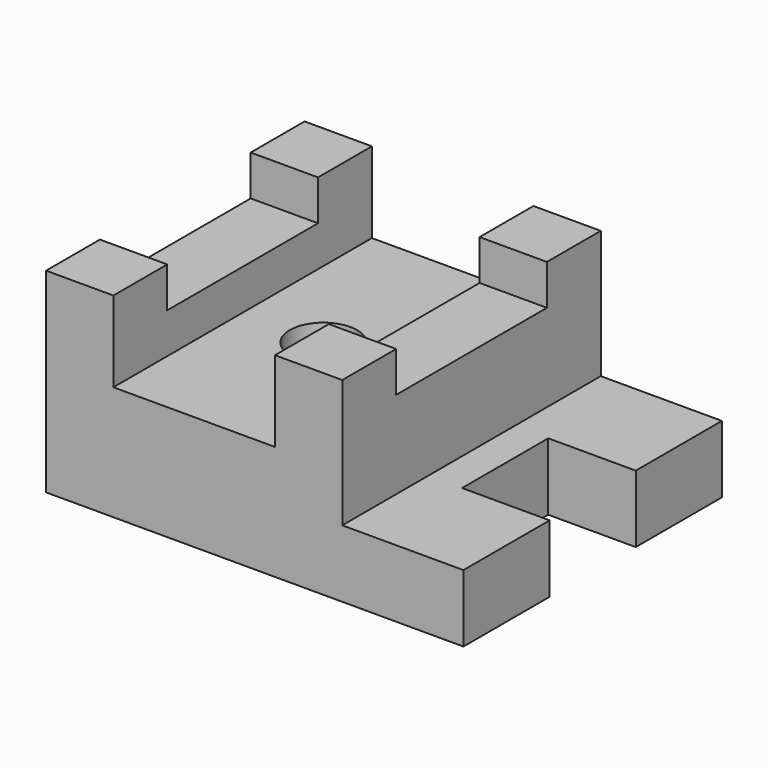
from build123d import *

# Parameters (mm, degrees)
F0_W     = 31.75
F0_H     = 31.75
F1_DEPTH = 92.075
F2_DEPTH = 31.75
F0_R     = 15.875
F3_DEPTH = 53.975
F0_H_2   = 88.9
F4_DEPTH = 73.025


# Not quite as in the source:
# - a feature names something its author has since deleted; it is built from what else it names


with BuildPart() as f1:
    # F0 (on Top) → F1 (new body)
    with BuildSketch(Plane.XY):
        with Locations((-53.975, 60.325)):
            Rectangle(F0_W, F0_H)
    extrude(amount=F1_DEPTH)



with BuildPart() as f1b:
    # F0 (on Top) → F1, piece 2 (new body)
    with BuildSketch(Plane.XY):
        with Locations((53.975, 60.325)):
            Rectangle(F0_W, F0_H)
    extrude(amount=F1_DEPTH)



with BuildPart() as f1c:
    # F0 (on Top) → F1, piece 3 (new body)
    with BuildSketch(Plane.XY):
        with Locations((53.975, -60.325)):
            Rectangle(F0_W, F0_H)
    extrude(amount=F1_DEPTH)


with BuildPart() as f1d:
    # F0 (on Top) → F1, piece 4 (new body)
    with BuildSketch(Plane.XY):
        with Locations((-53.975, -60.325)):
            Rectangle(F0_W, F0_H)
    extrude(amount=F1_DEPTH)


with BuildPart() as f1b_1:
    add(f1b.part)

    add(f1c.part)  # F2 merges F1c
    # F0 (on Top) → F2 (join)
    with BuildSketch(Plane.XY):
        Polygon((127, 25.4), (127, 76.2), (69.85, 76.2), (69.85, 44.45), (69.85, -44.45), (69.85, -76.2), (127, -76.2), (127, -25.4), (85.725, -25.4), (85.725, 25.4), align=None)
    extrude(amount=F2_DEPTH)


with BuildPart() as f1_1:
    add(f1.part)

    add(f1b_1.part)  # F3 merges F1b

    add(f1d.part)  # F3 merges F1d
    # F0 (on Top) → F3 (join)
    with BuildSketch(Plane.XY):
        Polygon((38.1, 44.45), (38.1, 76.2), (-38.1, 76.2), (-38.1, 44.45), (-38.1, -44.45), (-38.1, -76.2), (38.1, -76.2), (38.1, -44.45), align=None)
        Circle(F0_R, mode=Mode.SUBTRACT)
    extrude(amount=F3_DEPTH)

    # F0 (on Top) → F4 (join)
    with BuildSketch(Plane.XY):
        with Locations((-53.975, 0)):
            Rectangle(F0_W, F0_H_2)
        with Locations((53.975, 0)):
            Rectangle(F0_W, F0_H_2)
    extrude(amount=F4_DEPTH)


solid = f1_1.part
